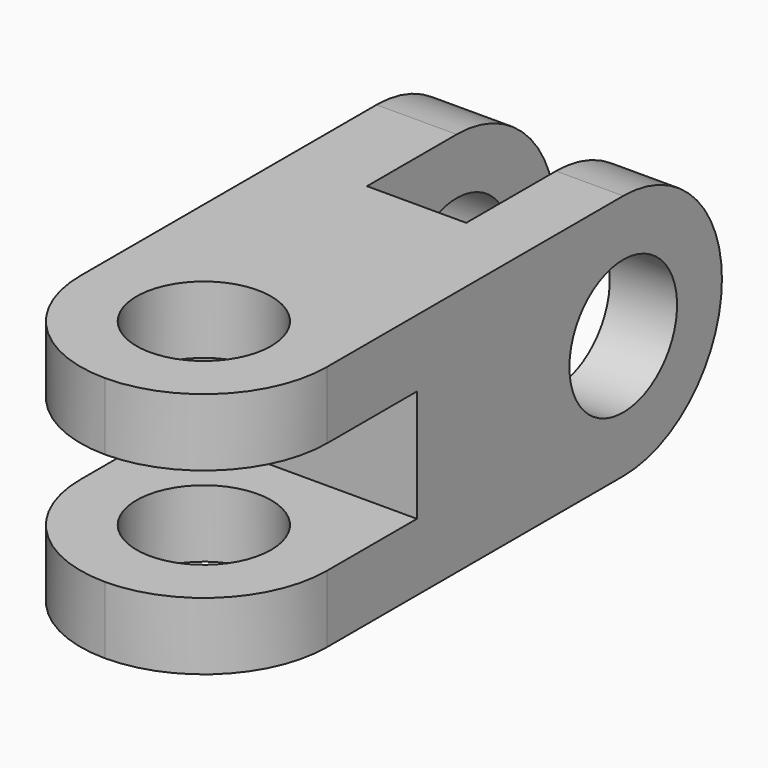
from build123d import *

# Parameters (mm, degrees)
F0_W      = 55.88
F0_H      = 55.88
F1_DEPTH  = 139.7
F2_R      = 27.93999
F3_W      = 22.4871877581
F3_H      = 35.5748719843
F3_H_2    = 25.40001
F4_DEPTH  = 55.881
F5_R      = 15.24
F6_DEPTH  = 55.881
F7_W      = 84.3253175833
F7_H      = 25.4
F8_DEPTH  = 55.881
F9_R      = 15.2425635054
F10_DEPTH = 55.881


# Not quite as in the source:
# - a fillet or chamfer is up to 0.001 mm smaller than in the source, because OpenCascade refuses the exact size
# - a feature names something its author has since deleted; it is built from what else it names


with BuildPart() as f1:
    # F0 (on Front) → F1 (new body)
    with BuildSketch(Plane.XZ):
        with Locations((27.94, -27.94)):
            Rectangle(F0_W, F0_H)
    extrude(amount=F1_DEPTH)

    # F2 (radius 27.94 in the source; OpenCascade refuses exactly that, so slightly less here)
    f2_edges = [f1.edges().sort_by_distance(p)[0] for p in [
        (0, -139.7, -27.94),
        (27.94, 0, 0),
        (27.94, 0, -55.88),
        (55.88, -139.7, -27.94),
    ]]
    fillet(f2_edges, radius=F2_R)

    # F3 (on face) → F4 (cut, through all)
    with BuildSketch(Plane(origin=(0, 0, -55.88), x_dir=(1, 0, 0), z_dir=(0, 0, -1))):
        with Locations((29.396406121, 10.1525540079)):
            Rectangle(F3_W, F3_H)
        with Locations((29.396406121, 40.639995)):
            Rectangle(F3_W, F3_H_2)
    extrude(amount=-F4_DEPTH, mode=Mode.SUBTRACT)

    # F5 (on face) → F6 (cut, through all)
    with BuildSketch(Plane(origin=(0, 0, 0), x_dir=(0, -1, 0), z_dir=(-1, 0, 0))):
        with Locations((27.94, -27.94)):
            Circle(F5_R)
    extrude(amount=-F6_DEPTH, mode=Mode.SUBTRACT)

    # F7 (on face) → F8 (cut, through all)
    with BuildSketch(Plane(origin=(0, 0, 0), x_dir=(0, -1, 0), z_dir=(-1, 0, 0))):
        with Locations((128.5226587916, -27.94)):
            Rectangle(F7_W, F7_H)
    extrude(amount=-F8_DEPTH, mode=Mode.SUBTRACT)

    # F9 (on face) → F10 (cut, through all)
    with BuildSketch(Plane(origin=(0, 0, -55.88), x_dir=(1, 0, 0), z_dir=(0, 0, -1))):
        with Locations((27.94, 111.76)):
            Circle(F9_R)
    extrude(amount=-F10_DEPTH, mode=Mode.SUBTRACT)


solid = f1.part
